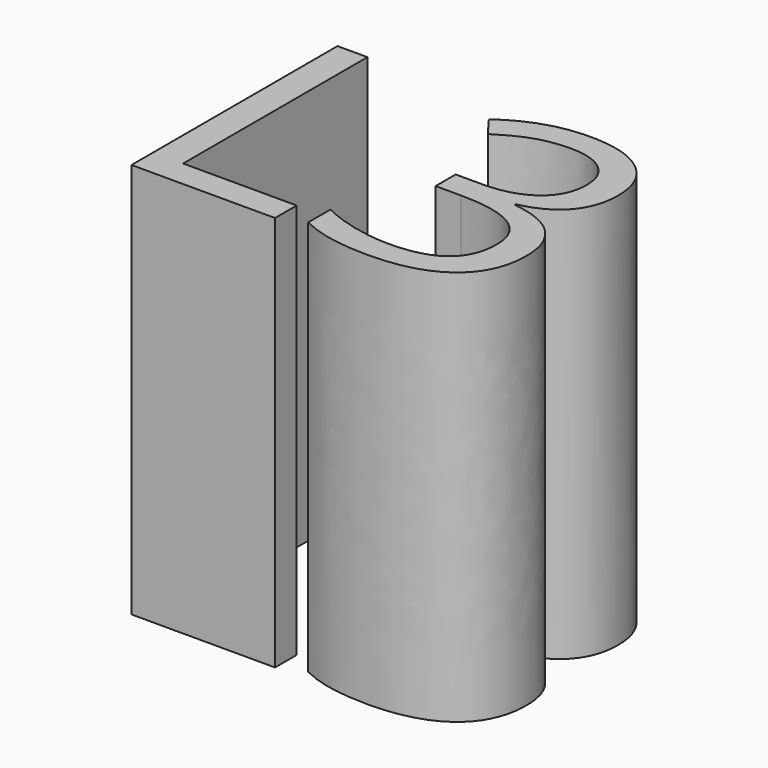
from build123d import *

# Parameters (mm, degrees)
F0_TEXT_SIZE = 9.115510611
F1_DEPTH     = 10


# Not quite as in the source:
# - Text() gives the source's letters only with a copy of the font that has no kerning and outlines rounded to 1/6400 em; it was checked with that copy


with BuildPart() as f1:
    # F0 (on Top) → F1 (new body)
    with BuildSketch(Plane.XY):
        with Locations((-5, -3.28158382)):
            Text('L3', F0_TEXT_SIZE, font='Open Sans', text_align=(TextAlign.LEFT, TextAlign.BOTTOM))
    extrude(amount=F1_DEPTH)


solid = f1.part
